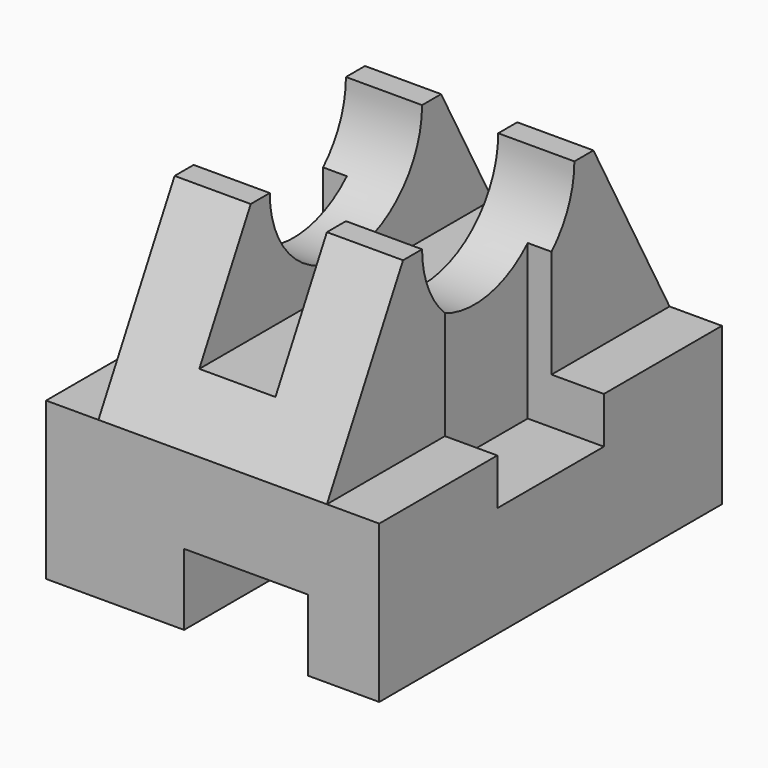
from build123d import *

# Parameters (mm, degrees)
F1_W      = 70
F1_H      = 90
F2_DEPTH  = 33
F3_W      = 26
F3_H      = 15
F4_DEPTH  = 90.001
F5_DEPTH  = 24
F6_W      = 16
F6_H      = 25
F7_DEPTH  = 90.001
F8_R      = 20
F9_DEPTH  = 59.001
F10_W     = 28
F10_H     = 50
F11_DEPTH = 16


# Not quite as in the source:
# - a pattern or mirror of a feature is missing from the dataset's text; its kind, count and spacing are read off the source's solid


with BuildPart() as f2:
    # F1 (on Top) → F2 (new body)
    with BuildSketch(Plane.XY):
        Rectangle(F1_W, F1_H)
    extrude(amount=-F2_DEPTH)

    # F3 (on face) → F4 (cut, through all)
    with BuildSketch(Plane.XZ.offset(45)):
        with Locations((7, -25.5)):
            Rectangle(F3_W, F3_H)
    extrude(amount=-F4_DEPTH, mode=Mode.SUBTRACT)

    # F0 (on Right) → F5 (join, symmetric)
    with BuildSketch(Plane.YZ):
        Polygon((-25, 37), (-45, 0), (45, 0), (25, 37), align=None)
    extrude(amount=F5_DEPTH, both=True)

    # F6 (on face) → F7 (cut, through all)
    with BuildSketch(Plane.XZ.offset(45)):
        with Locations((0, 24.5)):
            Rectangle(F6_W, F6_H)
    extrude(amount=-F7_DEPTH, mode=Mode.SUBTRACT)

    # F8 (on face) → F9 (cut, through all)
    with BuildSketch(Plane.YZ.offset(24)):
        with Locations((0, 37)):
            Circle(F8_R)
    extrude(amount=-F9_DEPTH, mode=Mode.SUBTRACT)

    # F10 (on face) → F11 (cut)
    with BuildSketch(Plane.YZ.offset(35)):
        with Locations((0, 15.2474023402)):
            Rectangle(F10_W, F10_H)
    f11 = extrude(amount=-F11_DEPTH, mode=Mode.SUBTRACT)

    # F11_copies: F11 across plane
    add(f11.mirror(Plane(origin=(0, 0, 0), x_dir=(0, 0, -1), z_dir=(-1, 0, 0))), mode=Mode.SUBTRACT)


solid = f2.part
